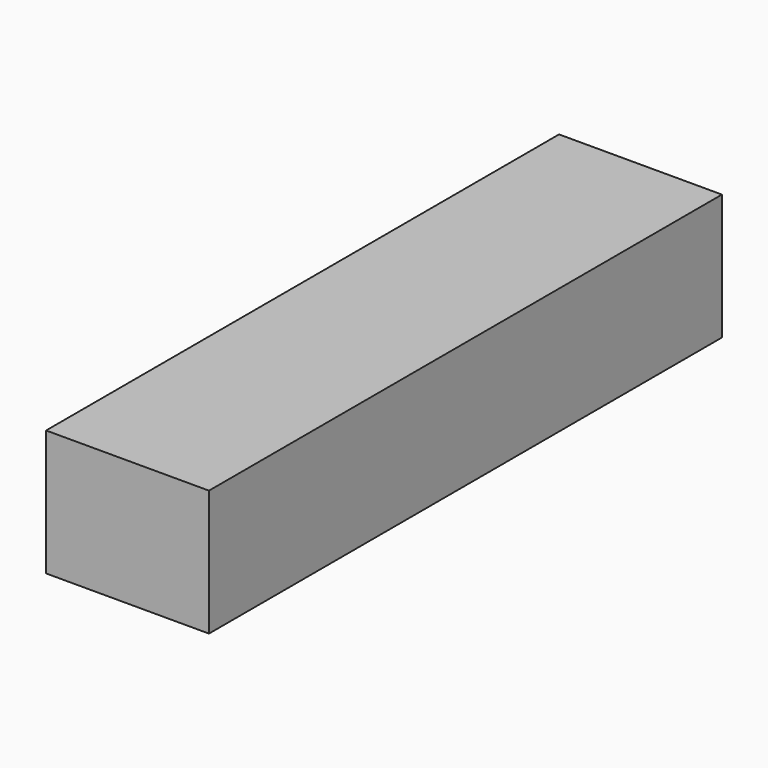
from build123d import *

# Parameters (mm, degrees)
F0_W          = 64.5265355706
F0_H          = 49.8596951365
F1_DEPTH      = 127
F1_DEPTH_BACK = 127


# Not quite as in the source:
# - a feature of the source that left no trace in its solid (it failed there, or was rolled back) is left out


with BuildPart() as f1:
    # F0 (on Front) → F1 (new body, two sides)
    with BuildSketch(Plane.XZ) as f1_sk:
        with Locations((-32.2632677853, 24.9298475683)):
            Rectangle(F0_W, F0_H)
    extrude(amount=F1_DEPTH)
    extrude(f1_sk.sketch, amount=-F1_DEPTH_BACK)


solid = f1.part
